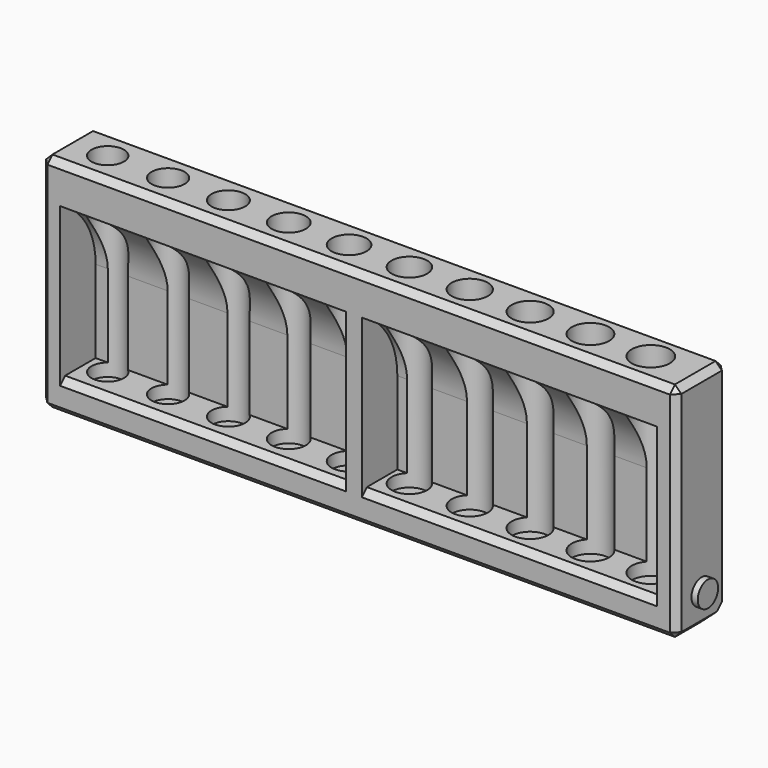
from build123d import *

# Parameters (mm, degrees)
F0_W          = 100
F0_H          = 10
F2_DEPTH      = 35
F3_START      = 3
F1_R          = 3
F1_R_2        = 2.95
F1_R_3        = 2.9
F1_R_4        = 2.85
F1_R_5        = 2.8
F1_R_6        = 2.75
F1_R_7        = 2.7
F1_R_8        = 2.65
F1_R_9        = 2.6
F1_R_10       = 2.55
F3_DEPTH      = 37
F5_START      = -3
F5_DEPTH      = 46.5
F6_START      = -52
F6_DEPTH      = 45
F7_SIZE       = 1
F8_R          = 2
F9_DEPTH      = 2
F9_DEPTH_BACK = 1
F10_START     = -99
F10_DEPTH     = 2
F11_T1_DEPTH  = 123


# Not quite as in the source:
# - a fillet or chamfer that OpenCascade refuses, or shapes differently, is made with other operations: its cross-section is extruded or revolved along the edge and cut away or added


with BuildPart() as f2:
    # F0 (on Top) → F2 (new body)
    with BuildSketch(Plane.XY):
        with Locations((-50, -5)):
            Rectangle(F0_W, F0_H)
    extrude(amount=F2_DEPTH)

    # F1 (on Top) → F3 (cut)
    with BuildSketch(Plane.XY.offset(F3_START)):
        with Locations((-8, -5)):
            Circle(F1_R)
        with Locations((-17.5, -5)):
            Circle(F1_R_2)
        with Locations((-27, -5)):
            Circle(F1_R_3)
        with Locations((-36.5, -5)):
            Circle(F1_R_4)
        with Locations((-46, -5)):
            Circle(F1_R_5)
        with Locations((-55.5, -5)):
            Circle(F1_R_6)
        with Locations((-65, -5)):
            Circle(F1_R_7)
        with Locations((-74.5, -5)):
            Circle(F1_R_8)
        with Locations((-84, -5)):
            Circle(F1_R_9)
        with Locations((-93.5, -5)):
            Circle(F1_R_10)
    extrude(amount=F3_DEPTH, mode=Mode.SUBTRACT)

    # F4 (on Right) → F5 (cut)
    with BuildSketch(Plane.YZ.offset(F5_START)):
        with BuildLine():
            Line((-13, 29.8321595662), (-13, 5))
            Line((-13, 5), (-3, 5))
            Line((-3, 5), (-3, 18))
            ThreePointArc((-3, 18), (-5.8348486101, 25.7459666924), (-13, 29.8321595662))
        make_face()
        with BuildLine():
            ThreePointArc((-15, 30), (-13.9964848766, 29.9579662735), (-13, 29.8321595662))
            Line((-13, 29.8321595662), (-13, 30))
            Line((-13, 30), (-15, 30))
        make_face()
    extrude(amount=-F5_DEPTH, mode=Mode.SUBTRACT)

    # F4 (on Right) → F6 (cut)
    with BuildSketch(Plane.YZ.offset(F6_START)):
        with BuildLine():
            Line((-13, 29.8321595662), (-13, 5))
            Line((-13, 5), (-3, 5))
            Line((-3, 5), (-3, 18))
            ThreePointArc((-3, 18), (-5.8348486101, 25.7459666924), (-13, 29.8321595662))
        make_face()
        with BuildLine():
            ThreePointArc((-15, 30), (-13.9964848766, 29.9579662735), (-13, 29.8321595662))
            Line((-13, 29.8321595662), (-13, 30))
            Line((-13, 30), (-15, 30))
        make_face()
    extrude(amount=-F6_DEPTH, mode=Mode.SUBTRACT)

    # F7
    f7_edges = [f2.edges().sort_by_distance(p)[0] for p in [
        (-50, -10, 35),
        (-100, -5, 35),
        (-50, 0, 35),
        (0, -5, 35),
        (0, -10, 17.5),
        (0, 0, 17.5),
        (0, -5, 0),
        (-50, -10, 0),
        (-100, -10, 17.5),
        (-74.5, -10, 5),
        (-26.25, -10, 5),
        (-100, -5, 0),
        (-100, 0, 17.5),
    ]]
    chamfer(f7_edges, length=F7_SIZE)

    # F8 (on Right) → F9 (join, two sides)
    with BuildSketch(Plane.YZ) as f9_sk:
        with Locations((-5, 5)):
            Circle(F8_R)
    extrude(amount=-F9_DEPTH)
    extrude(f9_sk.sketch, amount=F9_DEPTH_BACK)

    # F8 (on Right) → F10 (join)
    with BuildSketch(Plane.YZ.offset(F10_START)):
        with Locations((-5, 5)):
            Circle(F8_R)
    extrude(amount=-F10_DEPTH)

    # F11: fillet of radius 5 on 1 edges, made by hand

    # F11_s2 → F11_t1 (cut)
    with BuildSketch(Plane.YZ.offset(-111.5)):
        with BuildLine():
            ThreePointArc((0, 5), (-1.4644660941, 1.4644660941), (-5, 0))
            Line((-5, 0), (0, 0))
            Line((0, 0), (0, 5))
        make_face()
    extrude(amount=F11_T1_DEPTH, mode=Mode.SUBTRACT)


solid = f2.part
